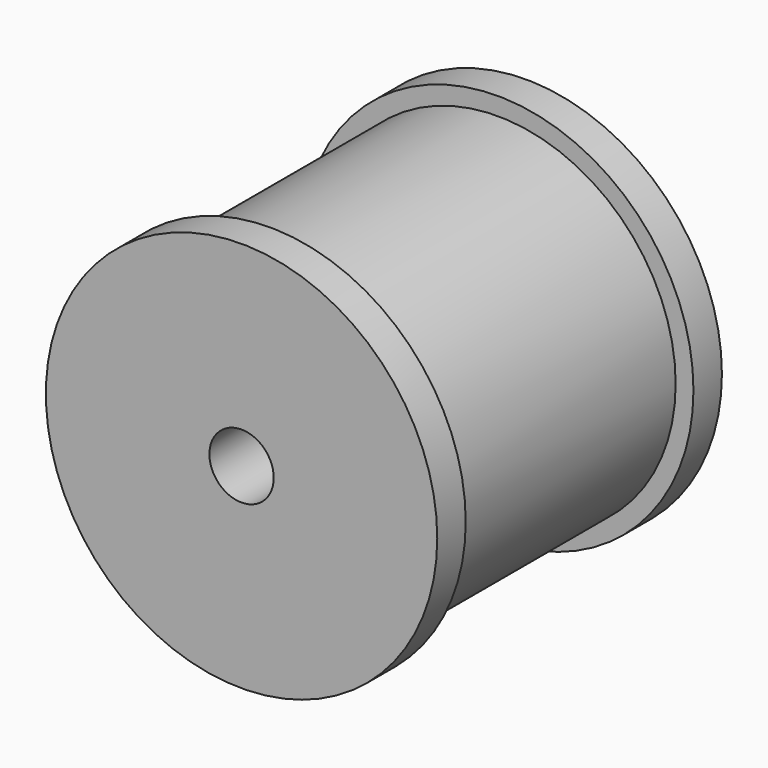
from build123d import *

# Parameters (mm, degrees)
F0_R     = 6.35
F1_DEPTH = 12.7
F2_R     = 6.985
F3_DEPTH = 1.27
F4_R     = 6.985
F5_DEPTH = 1.27
F6_R     = 1.14808
F7_DEPTH = 25.4


with BuildPart() as f1:
    # F0 (on Front) → F1 (new body)
    with BuildSketch(Plane.XZ):
        with Locations((-8.3881383762, 6.6514373757)):
            Circle(F0_R)
    extrude(amount=F1_DEPTH)

    # F2 (on face) → F3 (join)
    with BuildSketch(Plane.XZ.offset(12.7)):
        with Locations((-8.3881383762, 6.6514373757)):
            Circle(F2_R)
    extrude(amount=-F3_DEPTH)

    # F4 (on Front) → F5 (join)
    with BuildSketch(Plane.XZ):
        with Locations((-8.3881383762, 6.6514373757)):
            Circle(F4_R)
    extrude(amount=F5_DEPTH)

    # F6 (on face) → F7 (cut)
    with BuildSketch(Plane.XZ.offset(12.7)):
        with Locations((-8.3881383762, 6.6514373757)):
            Circle(F6_R)
    extrude(amount=-F7_DEPTH, mode=Mode.SUBTRACT)


solid = f1.part
